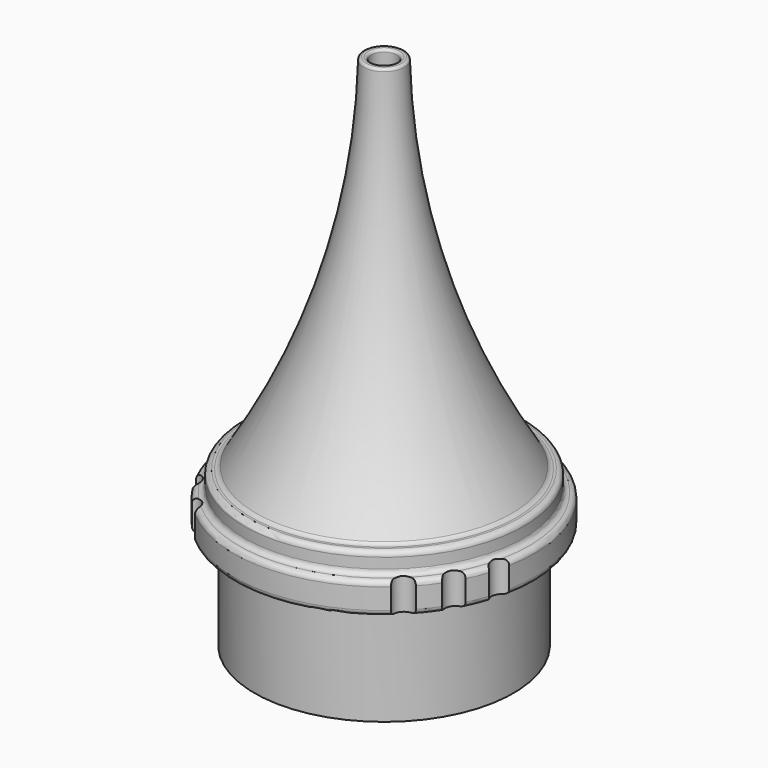
from build123d import *

# Parameters (mm, degrees)
F3_R     = 0.49999
F4_R     = 0.25
F5_R     = 1
F6_DEPTH = 25


# Not quite as in the source:
# - a fillet or chamfer is up to 0.001 mm smaller than in the source, because OpenCascade refuses the exact size


with BuildPart() as f2:
    # F0 (on Front) → F2 (revolve)
    with BuildSketch(Plane.XZ):
        with BuildLine():
            ThreePointArc((-1.95, 50), (-4.8099318339, 31.7720294528), (-12.5, 15))
            Line((-12.5, 15), (-13.5, 15))
            Line((-13.5, 15), (-13.5, 13))
            Line((-13.5, 13), (-14.5, 13))
            Line((-14.5, 13), (-14.5, 10))
            Line((-14.5, 10), (-12.5, 10))
            Line((-12.5, 10), (-12.5, 0))
            Line((-12.5, 0), (-10.5, 0))
            Line((-10.5, 0), (-10.5, 9))
            ThreePointArc((-10.5, 9), (-10.3714950106, 11.4743671533), (-9.913494827, 13.9093706798))
            ThreePointArc((-9.913494827, 13.9093706798), (-9.736621537, 14.4660116405), (-9.5, 15))
            ThreePointArc((-9.5, 15), (-3.2616783137, 32.0018598882), (-1.25, 50))
            Line((-1.25, 50), (-1.95, 50))
        make_face()
    revolve(axis=Axis((0, 0, 0), (0, 0, 1)))

    # F3 (radius 0.5 in the source; OpenCascade refuses exactly that, so slightly less here)
    f3_edges = [f2.edges().sort_by_distance(p)[0] for p in [
        (14.5, 0, 13),
        (14.5, 0, 10),
        (13.5, 0, 15),
        (12.5, 0, 15),
        (13.5, 0, 13),
    ]]
    fillet(f3_edges, radius=F3_R)

    # F4
    f4_edges = [f2.edges().sort_by_distance(p)[0] for p in [
        (1.95, 0, 50),
        (1.25, 0, 50),
    ]]
    fillet(f4_edges, radius=F4_R)

    # F5 (on Top) → F6 (cut)
    with BuildSketch(Plane.XY):
        with Locations((0, 14.8)):
            Circle(F5_R)
        with Locations((-3.9633087092, 14.2594594595)):
            Circle(F5_R)
        with Locations((3.9633087092, 14.2594594595)):
            Circle(F5_R)
        with Locations((-10.3673997816, -10.5620557549)):
            Circle(F5_R)
        with Locations((-12.817175976, -7.4)):
            Circle(F5_R)
        with Locations((-14.3307084907, -3.6974037046)):
            Circle(F5_R)
        with Locations((14.3307084907, -3.6974037046)):
            Circle(F5_R)
        with Locations((12.817175976, -7.4)):
            Circle(F5_R)
        with Locations((10.3673997816, -10.5620557549)):
            Circle(F5_R)
    extrude(amount=F6_DEPTH, mode=Mode.SUBTRACT)


solid = f2.part
